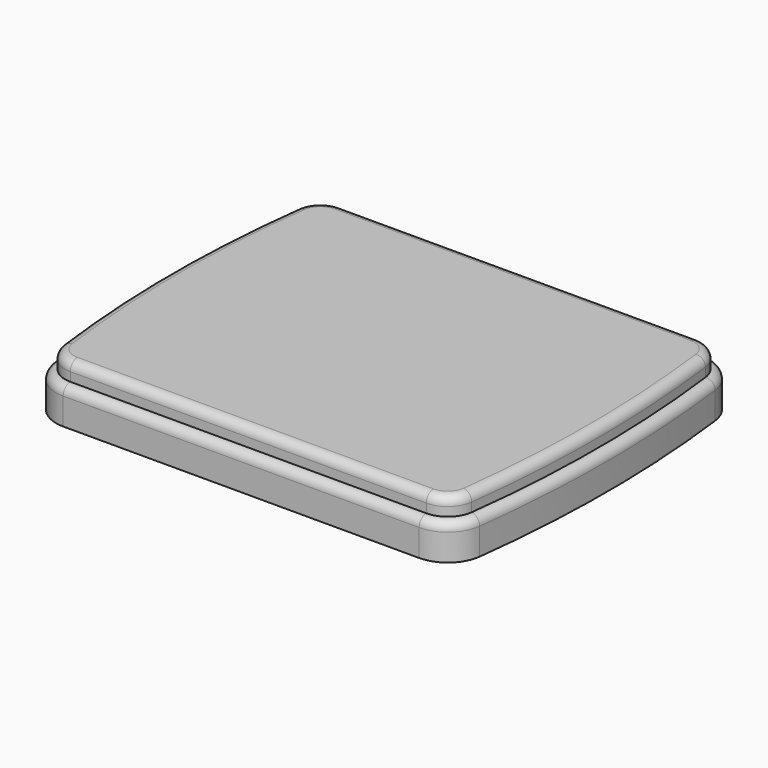
from build123d import *

# Parameters (mm, degrees)
F1_DEPTH = 2
F3_DEPTH = 1
F4_R     = 0.49999


# Not quite as in the source:
# - a fillet or chamfer is up to 0.001 mm smaller than in the source, because OpenCascade refuses the exact size
# - a feature names something its author has since deleted; it is built from what else it names


with BuildPart() as f1:
    # F0 (on Top) → F1 (new body)
    with BuildSketch(Plane.XY):
        with BuildLine():
            ThreePointArc((23.6934297445, 1.7622585683), (24.2075786729, 10), (23.6934297445, 18.2377414317))
            ThreePointArc((23.6934297445, 18.2377414317), (23.0323232276, 19.4886170119), (21.7089512216, 19.9890548979))
            Line((21.7089512216, 19.9890548979), (1.7932879128, 19.9890548979))
            ThreePointArc((1.7932879128, 19.9890548979), (0.4729381343, 19.491278737), (-0.1901730003, 18.2457313605))
            ThreePointArc((-0.1901730003, 18.2457313605), (-0.7214911689, 10), (-0.1901730003, 1.7542686395))
            ThreePointArc((-0.1901730003, 1.7542686395), (0.4729381343, 0.508721263), (1.7932879128, 0.0109451021))
            Line((1.7932879128, 0.0109451021), (21.7089512216, 0.0109451021))
            ThreePointArc((21.7089512216, 0.0109451021), (23.0323232276, 0.5113829881), (23.6934297445, 1.7622585683))
        make_face()
    extrude(amount=F1_DEPTH)

    # F2 (on face) → F3 (join)
    with BuildSketch(Plane.XY.offset(2)):
        with BuildLine():
            Line((21.7089512216, 19.4890548979), (1.7932879128, 19.4890548979))
            ThreePointArc((1.7932879128, 19.4890548979), (0.8030255789, 19.1157227772), (0.305692228, 18.1815622449))
            ThreePointArc((0.305692228, 18.1815622449), (-0.2214911689, 10), (0.305692228, 1.8184377551))
            ThreePointArc((0.305692228, 1.8184377551), (0.8030255789, 0.8842772228), (1.7932879128, 0.5109451021))
            Line((1.7932879128, 0.5109451021), (21.7089512216, 0.5109451021))
            ThreePointArc((21.7089512216, 0.5109451021), (22.7014802261, 0.8862735166), (23.1973101138, 1.8244302017))
            ThreePointArc((23.1973101138, 1.8244302017), (23.7075786729, 10), (23.1973101138, 18.1755697983))
            ThreePointArc((23.1973101138, 18.1755697983), (22.7014802261, 19.1137264834), (21.7089512216, 19.4890548979))
        make_face()
    extrude(amount=F3_DEPTH)

    # F4 (radius 0.5 in the source; OpenCascade refuses exactly that, so slightly less here)
    f4_edges = [f1.edges().sort_by_distance(p)[0] for p in [
        (11.75112, 0.010945, 2),
        (11.75112, 19.989055, 2),
        (23.032323, 0.511383, 2),
        (0.472938, 0.508721, 2),
        (24.207579, 10, 2),
        (-0.721491, 10, 2),
        (0.472938, 19.491279, 2),
        (23.032323, 19.488617, 2),
        (11.75112, 0.510945, 3),
        (0.803026, 0.884277, 3),
        (-0.221491, 10, 3),
        (11.75112, 19.489055, 3),
        (22.70148, 19.113726, 3),
        (23.707579, 10, 3),
        (0.803026, 19.115723, 3),
        (22.70148, 0.886274, 3),
    ]]
    fillet(f4_edges, radius=F4_R)


solid = f1.part
